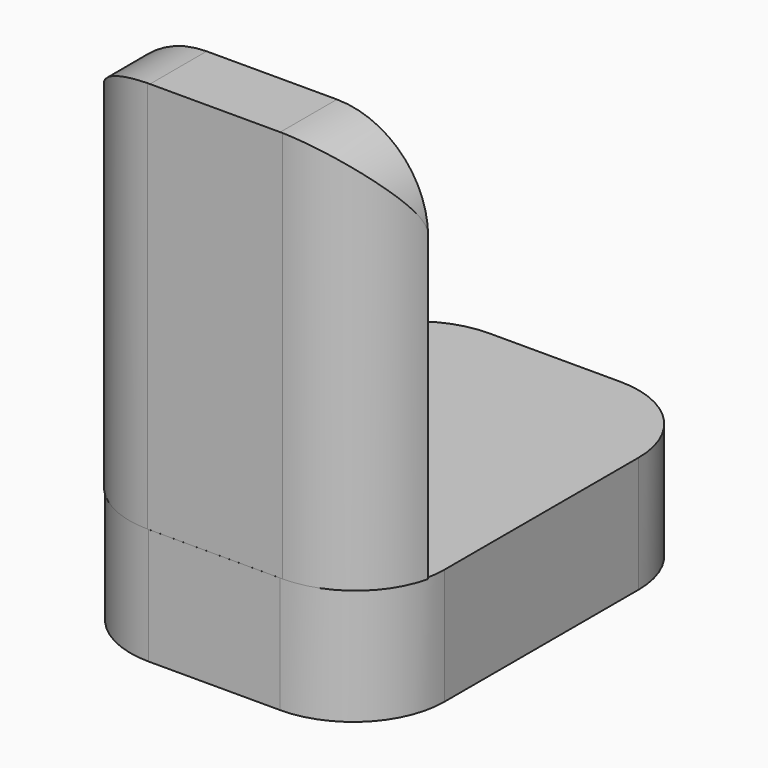
from build123d import *

# Parameters (mm, degrees)
F0_W          = 13.2919661701
F0_H          = 4.9218144268
F1_DEPTH      = 18
F2_W          = 13.2400542498
F2_H          = 16.6179258376
F3_DEPTH      = 3
F4_F1_R       = 3.8627416998
F4_F2_R       = 3.8627416998
F4_F3_R       = 3.8627416998
F4_F4_R       = 3.8627416998
F4_2_T1_DEPTH = 22.313708499
F4_2_T3_DEPTH = 35.4437393651


# Not quite as in the source:
# - a fillet or chamfer that OpenCascade refuses, or shapes differently, is made with other operations: its cross-section is extruded or revolved along the edge and cut away or added


with BuildPart() as f1:
    # F0 (on Front) → F1 (new body)
    with BuildSketch(Plane.XZ):
        with Locations((-30.6977089494, -34.0046109632)):
            Rectangle(F0_W, F0_H)
    extrude(amount=-F1_DEPTH)

    # F4: fillet of radius 3.8627416998 on 4 edges, made by hand

    # F4_f1
    f4_f1_edges = [f1.edges().sort_by_distance(p)[0] for p in [
        (-37.3436920345, 0, -34.0046109632),
    ]]
    fillet(f4_f1_edges, radius=F4_F1_R)

    # F4_f2
    f4_f2_edges = [f1.edges().sort_by_distance(p)[0] for p in [
        (-37.3436920345, 18, -34.0046109632),
    ]]
    fillet(f4_f2_edges, radius=F4_F2_R)

    # F4_f3
    f4_f3_edges = [f1.edges().sort_by_distance(p)[0] for p in [
        (-24.0517258644, 0, -34.0046109632),
    ]]
    fillet(f4_f3_edges, radius=F4_F3_R)

    # F4_f4
    f4_f4_edges = [f1.edges().sort_by_distance(p)[0] for p in [
        (-24.0517258644, 18, -34.0046109632),
    ]]
    fillet(f4_f4_edges, radius=F4_F4_R)


with BuildPart() as f3:
    # F2 (on Front) → F3 (new body)
    with BuildSketch(Plane.XZ):
        with Locations((-30.67163378, -23.2338802889)):
            Rectangle(F2_W, F2_H)
    extrude(amount=-F3_DEPTH)

    # F4#2: fillet of radius 3.8627416998 on 4 edges, made by hand

    # F4_2_s2 → F4_2_t1 (cut)
    with BuildSketch(Plane.XZ.offset(-12.6568542495)):
        with BuildLine():
            ThreePointArc((-24.0516066551, -18.7876590699), (-25.182977505, -16.05628822), (-27.9143483549, -14.9249173701))
            Line((-27.9143483549, -14.9249173701), (-24.0516066551, -14.9249173701))
            Line((-24.0516066551, -14.9249173701), (-24.0516066551, -18.7876590699))
        make_face()
        with BuildLine():
            ThreePointArc((-37.2916609049, -18.7876590699), (-36.160290055, -16.05628822), (-33.4289192051, -14.9249173701))
            Line((-33.4289192051, -14.9249173701), (-37.2916609049, -14.9249173701))
            Line((-37.2916609049, -14.9249173701), (-37.2916609049, -18.7876590699))
        make_face()
    extrude(amount=F4_2_T1_DEPTH, mode=Mode.SUBTRACT)

    # F4_2_s4 → F4_2_t3 (cut)
    with BuildSketch(Plane.XY.offset(-40.9557499714)):
        with BuildLine():
            ThreePointArc((-24.0516066551, 3), (-25.4096730705, 0.8417053065), (-27.8167693606, 0))
            Line((-27.8167693606, 0), (-24.0516066551, 0))
            Line((-24.0516066551, 0), (-24.0516066551, 3))
        make_face()
        with BuildLine():
            ThreePointArc((-37.2916609049, 3), (-35.9335944895, 0.8417053065), (-33.5264981994, 0))
            Line((-33.5264981994, 0), (-37.2916609049, 0))
            Line((-37.2916609049, 0), (-37.2916609049, 3))
        make_face()
    extrude(amount=F4_2_T3_DEPTH, mode=Mode.SUBTRACT)


solid = Compound([f1.part, f3.part])
